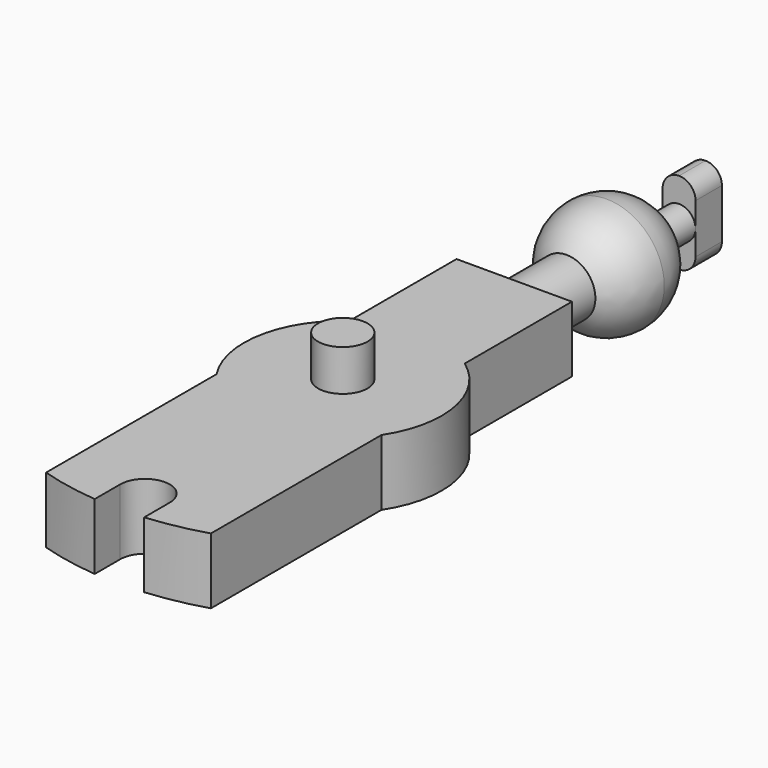
from build123d import *

# Parameters (mm, degrees)
F0_R          = 17
F1_DEPTH      = 2
F2_W          = 30
F2_H          = 30
F3_DEPTH      = 12.5
F4_W          = 30
F4_H          = 30
F5_DEPTH      = 12.5
F6_R          = 6
F7_DEPTH      = 2
F7_DEPTH_BACK = 2
F8_W          = 20
F8_H          = 5
F9_DEPTH      = 12.5
F10_R         = 1.5
F11_DEPTH     = 4.5
F15_R         = 1.75
F16_DEPTH     = 3.9689110868
F18_W         = 2
F18_H         = 5
F19_DEPTH     = 2
F20_R         = 0.99999
F21_R         = 1
F22_DEPTH     = 2.1458980338
F24_DEPTH     = 12.5


# Not quite as in the source:
# - a fillet or chamfer is up to 0.001 mm smaller than in the source, because OpenCascade refuses the exact size
# - a pattern or mirror of a feature is missing from the dataset's text; its kind, count and spacing are read off the source's solid


with BuildPart() as f1:
    # F0 (on Top) → F1 (new body, symmetric)
    with BuildSketch(Plane.XY):
        Circle(F0_R)
    extrude(amount=F1_DEPTH, both=True)

    # F2 (on Top) → F3 (cut, symmetric)
    with BuildSketch(Plane.XY):
        with Locations((20, -15)):
            Rectangle(F2_W, F2_H)
    f3 = extrude(amount=F3_DEPTH, both=True, mode=Mode.SUBTRACT)

    # F3_copies: F3 across plane
    add(f3.mirror(Plane(origin=(0, 0, 0), x_dir=(0, 0, -1), z_dir=(-1, 0, 0))), mode=Mode.SUBTRACT)

    # F4 (on Top) → F5 (cut, symmetric)
    with BuildSketch(Plane.XY):
        with Locations((18.5, 15)):
            Rectangle(F4_W, F4_H)
    f5 = extrude(amount=F5_DEPTH, both=True, mode=Mode.SUBTRACT)

    # F5_copies: F5 across plane
    add(f5.mirror(Plane(origin=(0, 0, 0), x_dir=(0, 0, -1), z_dir=(-1, 0, 0))), mode=Mode.SUBTRACT)

    # F6 (on Top) → F7 (join, two sides)
    with BuildSketch(Plane.XY) as f7_sk:
        Circle(F6_R)
    extrude(amount=F7_DEPTH)
    extrude(f7_sk.sketch, amount=-F7_DEPTH_BACK)

    # F8 (on Top) → F9 (cut, symmetric)
    with BuildSketch(Plane.XY):
        with Locations((0, 15.5)):
            Rectangle(F8_W, F8_H)
    extrude(amount=F9_DEPTH, both=True, mode=Mode.SUBTRACT)

    # F10 (on Top) → F11 (join, symmetric)
    with BuildSketch(Plane.XY):
        Circle(F10_R)
    extrude(amount=F11_DEPTH, both=True)



with BuildPart() as f13:
    # F12 (on Top) → F13 (revolve)
    with BuildSketch(Plane.XY):
        with BuildLine():
            ThreePointArc((0, 16.5), (2.4748737342, 17.5251262658), (3.5, 20))
            ThreePointArc((3.5, 20), (2.4748737342, 22.4748737342), (0, 23.5))
            Line((0, 23.5), (0, 16.5))
        make_face()
    revolve(axis=Axis((0, 19.7940547951, 0), (0, 1, 0)))


with BuildPart() as f1_1:
    add(f1.part)

    add(f13.part)  # F16 merges F13
    # F15 (on offset) → F16 (join, through all)
    with BuildSketch(Plane.XZ.offset(-13)):
        Circle(F15_R)
    extrude(amount=-F16_DEPTH)



with BuildPart() as f19:
    # F18 (on offset) → F19 (new body)
    with BuildSketch(Plane.XZ.offset(-25.5)):
        Rectangle(F18_W, F18_H)
    extrude(amount=-F19_DEPTH)

    # F20 (radius 1 in the source; OpenCascade refuses exactly that, so slightly less here)
    f20_edges = [f19.edges().sort_by_distance(p)[0] for p in [
        (1, 26.5, 2.5),
        (-1, 26.5, 2.5),
        (-1, 26.5, -2.5),
        (1, 26.5, -2.5),
    ]]
    fillet(f20_edges, radius=F20_R)


with BuildPart() as f1_2:
    add(f1_1.part)

    add(f19.part)  # F22 merges F19
    # F21 (on offset) → F22 (join, through all)
    with BuildSketch(Plane.XZ.offset(-25.5)):
        Circle(F21_R)
    extrude(amount=F22_DEPTH)

    # F23 (on Top) → F24 (cut, symmetric)
    with BuildSketch(Plane.XY):
        with BuildLine():
            Line((-1.5, -15), (-1.5, -20))
            Line((-1.5, -20), (1.5, -20))
            Line((1.5, -20), (1.5, -15))
            ThreePointArc((1.5, -15), (0, -13.5), (-1.5, -15))
        make_face()
    extrude(amount=F24_DEPTH, both=True, mode=Mode.SUBTRACT)


solid = f1_2.part
